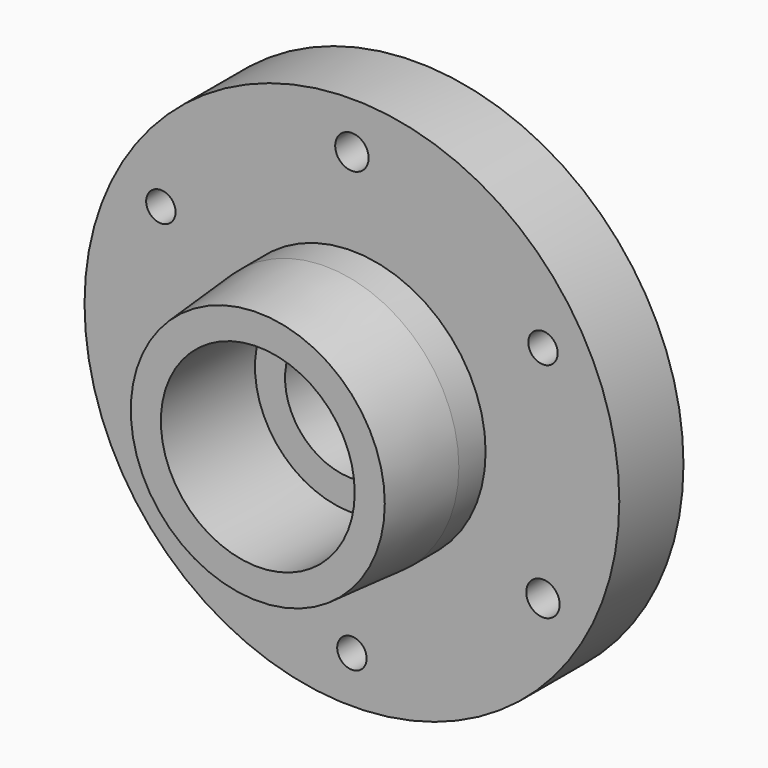
from build123d import *

# Parameters (mm, degrees)
F0_R            = 200
F0_R_2          = 100
F0_R_3          = 72.5
F0_R_4          = 50
F1_DEPTH        = 30
F2_DEPTH        = 118
F3_DEPTH        = 30
F5_D            = 25
F5_CBORE_D      = 51
F5_CBORE_DEPTH  = 10
F5_COPIES_COUNT = 3
F6_D            = 22
F6_COPIES_COUNT = 3
F7_SIZE2        = 63
F7_SIZE         = 5


# Not quite as in the source:
# - a pattern or mirror of a feature is missing from the dataset's text; its kind, count and spacing are read off the source's solid


with BuildPart() as f1:
    # F0 (on Front) → F1 (new body)
    with BuildSketch(Plane.XZ):
        Circle(F0_R)
        Circle(F0_R_2, mode=Mode.SUBTRACT)
        Circle(F0_R_2)
        Circle(F0_R_3, mode=Mode.SUBTRACT)
        Circle(F0_R_3)
        Circle(F0_R_4, mode=Mode.SUBTRACT)
    extrude(amount=F1_DEPTH)

    # F0 (on Front) → F2 (join)
    with BuildSketch(Plane.XZ):
        Circle(F0_R_2)
        Circle(F0_R_3, mode=Mode.SUBTRACT)
    extrude(amount=F2_DEPTH)

    # F0 (on Front) → F3 (join)
    with BuildSketch(Plane.XZ):
        Circle(F0_R)
        Circle(F0_R_2, mode=Mode.SUBTRACT)
    extrude(amount=-F3_DEPTH)

    # F5 (through all)
    with Locations(Plane(origin=(0, 30, 0), x_dir=(-1, 0, 0), z_dir=(0, 1, 0))):
        with Locations((0, 165)):
            f5 = CounterBoreHole(F5_D / 2, F5_CBORE_D / 2, F5_CBORE_DEPTH)

    # F5_copies: F5 ×3 about axis
    f5_copies_axis = Axis((0, 0, 0), (0, 1, 0))
    for i in range(1, F5_COPIES_COUNT):
        add(f5.rotate(f5_copies_axis, i * 360 / F5_COPIES_COUNT), mode=Mode.SUBTRACT)

    # F6 (through all)
    with Locations(Plane(origin=(0, 30, 0), x_dir=(-1, 0, 0), z_dir=(0, 1, 0))):
        with Locations((-142.8941916244, 82.5)):
            f6 = Hole(F6_D / 2)

    # F6_copies: F6 ×3 about axis
    f6_copies_axis = Axis((0, 0, 0), (0, 1, 0))
    for i in range(1, F6_COPIES_COUNT):
        add(f6.rotate(f6_copies_axis, i * 360 / F6_COPIES_COUNT), mode=Mode.SUBTRACT)

    # F7
    f7_edges = [f1.edges().sort_by_distance(p)[0] for p in [
        (-100, -118, 0),
    ]]
    f7_side = f1.faces().sort_by_distance((-97.171573, -118, 0))[0]
    chamfer(f7_edges, length=F7_SIZE, length2=F7_SIZE2, reference=f7_side)


solid = f1.part
